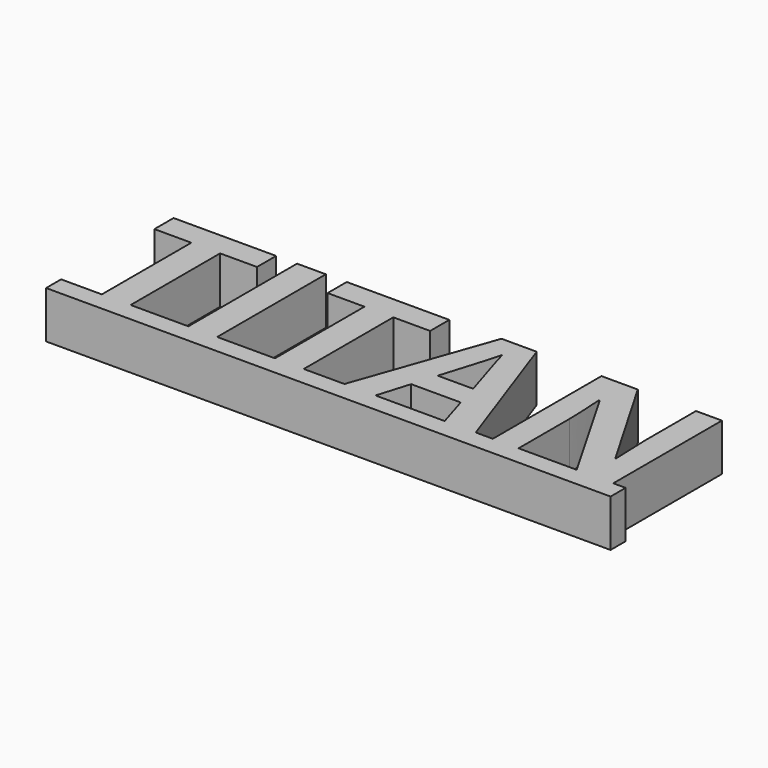
from build123d import *

# Parameters (mm, degrees)
F0_TEXT_SIZE = 20.2211690363
F1_DEPTH     = 5


# Not quite as in the source:
# - Text() gives the source's letters only with a copy of the font that has no kerning and outlines rounded to 1/6400 em; it was checked with that copy


with BuildPart() as f1:
    # F0 (on Top) → F1 (new body)
    with BuildSketch(Plane.XY):
        Polygon((13.8397265438, -3.0785273304), (9.5142921046, -3.0785273304), (9.5142921046, -5.0785273304), (69.5142921046, -5.0785273304), (69.5142921046, -3.0785273304), (68.2030756749, -3.0785273304), (64.3136601931, -3.0785273304), (58.1335654064, -3.0785273304), (55.3973884711, -3.0785273304), (53.5806428155, -3.0785273304), (50.2820646165, -3.0785273304), (42.9266143795, -3.0785273304), (39.6280361805, -3.0785273304), (35.3057612989, -3.0785273304), (32.2441499245, -3.0785273304), (26.1019698297, -3.0785273304), (23.0403584553, -3.0785273304), (16.9013379182, -3.0785273304), align=None)
        with Locations((9.5142921046, -3.0785273304)):
            Text('TITAN', F0_TEXT_SIZE, font='Open Sans', font_style=FontStyle.BOLD, text_align=(TextAlign.LEFT, TextAlign.BOTTOM))
    extrude(amount=F1_DEPTH)


solid = f1.part
